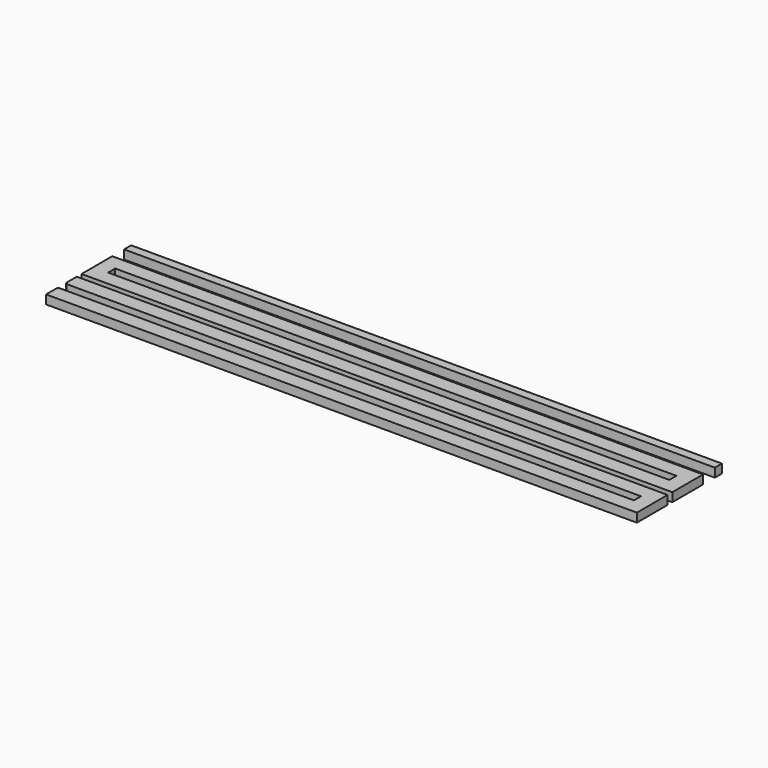
from build123d import *

# Parameters (mm, degrees)
F0_W     = 200
F0_H     = 3
F1_DEPTH = 3
F0_H_2   = 13
F0_W_2   = 190
F3_DEPTH = 25
F4_SIZE  = 0.5


with BuildPart() as f1:
    # F0 (on Top) → F1 (new body)
    with BuildSketch(Plane.XY):
        with Locations((0, 22.59805426)):
            Rectangle(F0_W, F0_H)
    extrude(amount=F1_DEPTH)


with BuildPart() as f1b:
    # F0 (on Top) → F1, piece 2 (new body)
    with BuildSketch(Plane.XY):
        with Locations((0, 9.599968791)):
            Rectangle(F0_W, F0_H_2)
        with Locations((0, 9.599968791)):
            Rectangle(F0_W_2, F0_H, mode=Mode.SUBTRACT)
    extrude(amount=F1_DEPTH)


with BuildPart() as f2_1:
    # F2: copy of F1b
    add(f1b.part.moved(Location((0, -15, 0))))

    # F3 (cut): a face of the model
    f3_faces = [f2_1.faces().sort_by_distance(p)[0] for p in [
        (-95, -5.400031209, 1.5),
    ]]
    extrude(f3_faces, amount=-F3_DEPTH, mode=Mode.SUBTRACT)

    # F4
    f4_edges = [f2_1.edges().sort_by_distance(p)[0] for p in [
        (-100, -3.900031, 1.5),
        (-100, -6.900031, 1.5),
    ]]
    chamfer(f4_edges, length=F4_SIZE)


solid = Compound([f1.part, f1b.part, f2_1.part])
